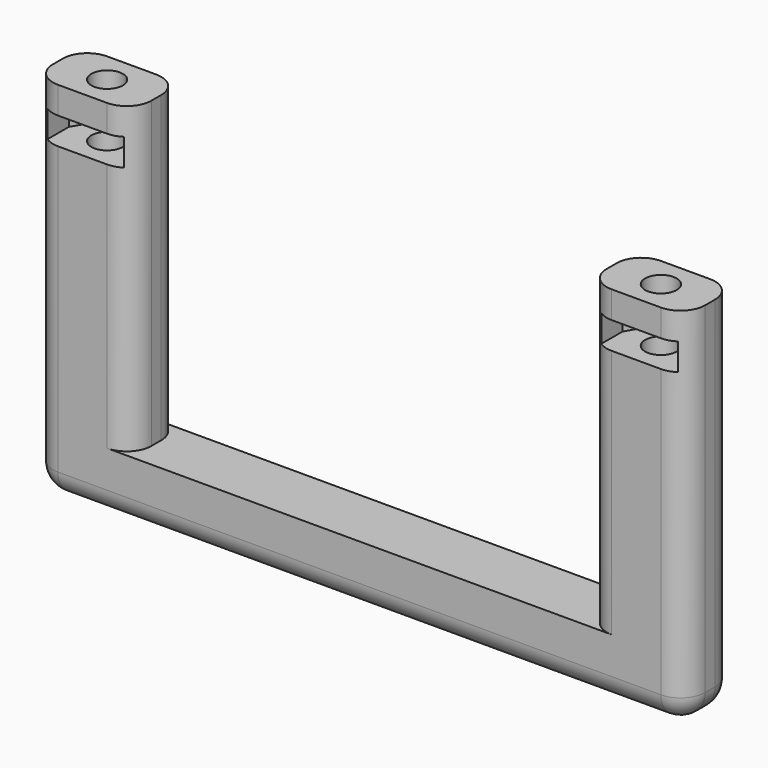
from build123d import *

# Parameters (mm, degrees)
F0_W         = 5.2
F0_H         = 2
F1_DEPTH     = 2.5
F3_DEPTH     = 2.2
F4_W         = 8
F4_H         = 5
F5_DEPTH     = 2.2
F6_R         = 1.28
F7_DEPTH     = 25
F8_T1_DEPTH  = 1
F8_T3_DEPTH  = 49
F8_T5_DEPTH  = 29.7
F8_T7_DEPTH  = 32.7
F8_S11_W     = 2
F8_S11_H     = 2
F8_T12_DEPTH = 2
F8_S17_W     = 2
F8_S17_H     = 2
F8_T18_DEPTH = 2
F8_S23_W     = 2
F8_S23_H     = 2
F8_T24_DEPTH = 2
F8_S29_W     = 2
F8_S29_H     = 2
F8_T30_DEPTH = 2


# Not quite as in the source:
# - a fillet or chamfer that OpenCascade refuses, or shapes differently, is made with other operations: its cross-section is extruded or revolved along the edge and cut away or added


with BuildPart() as f1:
    # F0 (on Front) → F1 (new body, symmetric)
    with BuildSketch(Plane.XZ):
        Polygon((18.5, 0), (0, 0), (0, -5), (26.5, -5), (26.5, 0), (22.5, 0), align=None)
        Polygon((18.5, 22.5), (18.5, 0), (22.5, 0), (26.5, 0), (26.5, 22.5), (25.1, 22.5), (25.1, 20.5), (19.9, 20.5), (19.9, 22.5), align=None)
        with Locations((22.5, 21.5)):
            Rectangle(F0_W, F0_H)
        Polygon((0, -5), (0, 0), (-18.5, 0), (-22.5, 0), (-26.5, 0), (-26.5, -5), align=None)
        Polygon((-22.5, 0), (-18.5, 0), (-18.5, 22.5), (-19.9, 22.5), (-19.9, 20.5), (-25.1, 20.5), (-25.1, 22.5), (-26.5, 22.5), (-26.5, 0), align=None)
        with Locations((-22.5, 21.5)):
            Rectangle(F0_W, F0_H)
    extrude(amount=F1_DEPTH, both=True)

    # F2 (on face) → F3 (cut)
    with BuildSketch(Plane.XY.offset(22.5)):
        Polygon((19.3823289357, -2.5), (20.8312208665, -2.5), (19.3823289357, -0.011275415), align=None)
        Polygon((20.8312208665, -2.5), (24.1798700484, -2.5), (25.6176710643, 0.011275415), (24.1687791335, 2.5), (20.8201299516, 2.5), (19.3823289357, -0.011275415), align=None)
        Polygon((24.068600328, -2.6943446348), (24.1798700484, -2.5), (20.8312208665, -2.5), (20.9509292637, -2.7056200498), align=None)
        Polygon((24.1798700484, -2.5), (25.6176710643, -2.5), (25.6176710643, 0.011275415), align=None)
        Polygon((-24.1798700484, -2.5), (-20.8312208665, -2.5), (-19.3823289357, -0.011275415), (-20.8201299516, 2.5), (-24.1687791335, 2.5), (-25.6176710643, 0.011275415), align=None)
        Polygon((-20.9509292637, -2.7056200498), (-20.8312208665, -2.5), (-24.1798700484, -2.5), (-24.068600328, -2.6943446348), align=None)
        Polygon((-25.6176710643, -2.5), (-24.1798700484, -2.5), (-25.6176710643, 0.011275415), align=None)
        Polygon((-20.8312208665, -2.5), (-19.3823289357, -2.5), (-19.3823289357, -0.011275415), align=None)
    extrude(amount=-F3_DEPTH, mode=Mode.SUBTRACT)

    # F4 (on face) → F5 (join)
    with BuildSketch(Plane.XY.offset(22.5)):
        with Locations((-22.5, 0)):
            Rectangle(F4_W, F4_H)
        Polygon((25.6176710643, 0.011275415), (24.1687791335, 2.5), (18.5, 2.5), (18.5, -2.5), (25.6176710643, -2.5), align=None)
        Polygon((26.5, -2.5), (26.5, 2.5), (24.1687791335, 2.5), (25.6176710643, 0.011275415), (25.6176710643, -2.5), align=None)
    extrude(amount=F5_DEPTH)

    # F6 (on face) → F7 (cut)
    with BuildSketch(Plane.XY.offset(24.7)):
        with Locations((-22.5, 0)):
            Circle(F6_R)
        with Locations((22.5, 0)):
            Circle(F6_R)
    extrude(amount=-F7_DEPTH, mode=Mode.SUBTRACT)

    # F8: fillet of radius 2 on 12 edges, made by hand

    # F8_s2 → F8_t1 (cut)
    with BuildSketch(Plane.XZ.offset(-0.5)):
        with BuildLine():
            ThreePointArc((-26.5, -3), (-25.9142135624, -4.4142135624), (-24.5, -5))
            Line((-24.5, -5), (-26.5, -5))
            Line((-26.5, -5), (-26.5, -3))
        make_face()
        with BuildLine():
            ThreePointArc((24.5, -5), (25.9142135624, -4.4142135624), (26.5, -3))
            Line((26.5, -3), (26.5, -5))
            Line((26.5, -5), (24.5, -5))
        make_face()
    extrude(amount=F8_T1_DEPTH, mode=Mode.SUBTRACT)

    # F8_s4 → F8_t3 (cut)
    with BuildSketch(Plane.YZ.offset(-24.5)):
        with BuildLine():
            ThreePointArc((2.5, -3), (1.9142135624, -4.4142135624), (0.5, -5))
            Line((0.5, -5), (2.5, -5))
            Line((2.5, -5), (2.5, -3))
        make_face()
        with BuildLine():
            ThreePointArc((-2.5, -3), (-1.9142135624, -4.4142135624), (-0.5, -5))
            Line((-0.5, -5), (-2.5, -5))
            Line((-2.5, -5), (-2.5, -3))
        make_face()
    extrude(amount=F8_T3_DEPTH, mode=Mode.SUBTRACT)

    # F8_s6 → F8_t5 (cut)
    with BuildSketch(Plane.XY):
        with BuildLine():
            ThreePointArc((20.5, -2.5), (19.0857864376, -1.9142135624), (18.5, -0.5))
            Line((18.5, -0.5), (18.5, -2.5))
            Line((18.5, -2.5), (20.5, -2.5))
        make_face()
        with BuildLine():
            ThreePointArc((20.5, 2.5), (19.0857864376, 1.9142135624), (18.5, 0.5))
            Line((18.5, 0.5), (18.5, 2.5))
            Line((18.5, 2.5), (20.5, 2.5))
        make_face()
        with BuildLine():
            ThreePointArc((-18.5, -0.5), (-19.0857864376, -1.9142135624), (-20.5, -2.5))
            Line((-20.5, -2.5), (-18.5, -2.5))
            Line((-18.5, -2.5), (-18.5, -0.5))
        make_face()
        with BuildLine():
            ThreePointArc((-20.5, 2.5), (-19.0857864376, 1.9142135624), (-18.5, 0.5))
            Line((-18.5, 0.5), (-18.5, 2.5))
            Line((-18.5, 2.5), (-20.5, 2.5))
        make_face()
    extrude(amount=F8_T5_DEPTH, mode=Mode.SUBTRACT)

    # F8_s8 → F8_t7 (cut)
    with BuildSketch(Plane.XY.offset(-3)):
        with BuildLine():
            ThreePointArc((24.5, -2.5), (25.9142135624, -1.9142135624), (26.5, -0.5))
            Line((26.5, -0.5), (26.5, -2.5))
            Line((26.5, -2.5), (24.5, -2.5))
        make_face()
        with BuildLine():
            ThreePointArc((24.5, 2.5), (25.9142135624, 1.9142135624), (26.5, 0.5))
            Line((26.5, 0.5), (26.5, 2.5))
            Line((26.5, 2.5), (24.5, 2.5))
        make_face()
        with BuildLine():
            ThreePointArc((-24.5, -2.5), (-25.9142135624, -1.9142135624), (-26.5, -0.5))
            Line((-26.5, -0.5), (-26.5, -2.5))
            Line((-26.5, -2.5), (-24.5, -2.5))
        make_face()
        with BuildLine():
            ThreePointArc((-24.5, 2.5), (-25.9142135624, 1.9142135624), (-26.5, 0.5))
            Line((-26.5, 0.5), (-26.5, 2.5))
            Line((-26.5, 2.5), (-24.5, 2.5))
        make_face()
    extrude(amount=F8_T7_DEPTH, mode=Mode.SUBTRACT)


with BuildPart() as f8_tool10:
    # F8_s11 → F8_t12 (new body)
    with BuildSketch(Plane.XZ.offset(-0.5)):
        with Locations((-25.5, -4)):
            Rectangle(F8_S11_W, F8_S11_H)
    extrude(amount=-F8_T12_DEPTH)

    # F8_s13 → F8_t14 (revolve, cut)
    with BuildSketch(Plane(origin=(-24.5, 0.5, -3), x_dir=(0.7071067812, 0, 0.7071067812), z_dir=(-0.7071067812, 0, 0.7071067812))):
        with BuildLine():
            ThreePointArc((0, -2), (2, 0), (0, 2))
            Line((0, 2), (0, -2))
        make_face()
    revolve(axis=Axis((-24.5, 0.5, -3), (0, 1, 0)), mode=Mode.SUBTRACT)


with BuildPart() as f1_1:
    add(f1.part)

    # F8_t9: cut F8_tool10
    add(f8_tool10.part, mode=Mode.SUBTRACT)


with BuildPart() as f8_tool16:
    # F8_s17 → F8_t18 (new body)
    with BuildSketch(Plane.XZ.offset(0.5)):
        with Locations((-25.5, -4)):
            Rectangle(F8_S17_W, F8_S17_H)
    extrude(amount=F8_T18_DEPTH)

    # F8_s19 → F8_t20 (revolve, cut)
    with BuildSketch(Plane(origin=(-24.5, -0.5, -3), x_dir=(0.7071067812, 0, 0.7071067812), z_dir=(0.7071067812, 0, -0.7071067812))):
        with BuildLine():
            ThreePointArc((0, -2), (2, 0), (0, 2))
            Line((0, 2), (0, -2))
        make_face()
    revolve(axis=Axis((-24.5, -0.5, -3), (0, -1, 0)), mode=Mode.SUBTRACT)


with BuildPart() as f1_2:
    add(f1_1.part)

    # F8_t15: cut F8_tool16
    add(f8_tool16.part, mode=Mode.SUBTRACT)


with BuildPart() as f8_tool22:
    # F8_s23 → F8_t24 (new body)
    with BuildSketch(Plane.YZ.offset(24.5)):
        with Locations((1.5, -4)):
            Rectangle(F8_S23_W, F8_S23_H)
    extrude(amount=F8_T24_DEPTH)

    # F8_s25 → F8_t26 (revolve, cut)
    with BuildSketch(Plane(origin=(24.5, 0.5, -3), x_dir=(0, -0.7071067812, 0.7071067812), z_dir=(0, 0.7071067812, 0.7071067812))):
        with BuildLine():
            ThreePointArc((0, -2), (2, 0), (0, 2))
            Line((0, 2), (0, -2))
        make_face()
    revolve(axis=Axis((24.5, 0.5, -3), (1, 0, 0)), mode=Mode.SUBTRACT)


with BuildPart() as f1_3:
    add(f1_2.part)

    # F8_t21: cut F8_tool22
    add(f8_tool22.part, mode=Mode.SUBTRACT)


with BuildPart() as f8_tool28:
    # F8_s29 → F8_t30 (new body)
    with BuildSketch(Plane.YZ.offset(24.5)):
        with Locations((-1.5, -4)):
            Rectangle(F8_S29_W, F8_S29_H)
    extrude(amount=F8_T30_DEPTH)

    # F8_s31 → F8_t32 (revolve, cut)
    with BuildSketch(Plane(origin=(24.5, -0.5, -3), x_dir=(0, 0.7071067812, 0.7071067812), z_dir=(0, 0.7071067812, -0.7071067812))):
        with BuildLine():
            ThreePointArc((0, -2), (2, 0), (0, 2))
            Line((0, 2), (0, -2))
        make_face()
    revolve(axis=Axis((24.5, -0.5, -3), (1, 0, 0)), mode=Mode.SUBTRACT)


with BuildPart() as f1_4:
    add(f1_3.part)

    # F8_t27: cut F8_tool28
    add(f8_tool28.part, mode=Mode.SUBTRACT)


solid = f1_4.part
